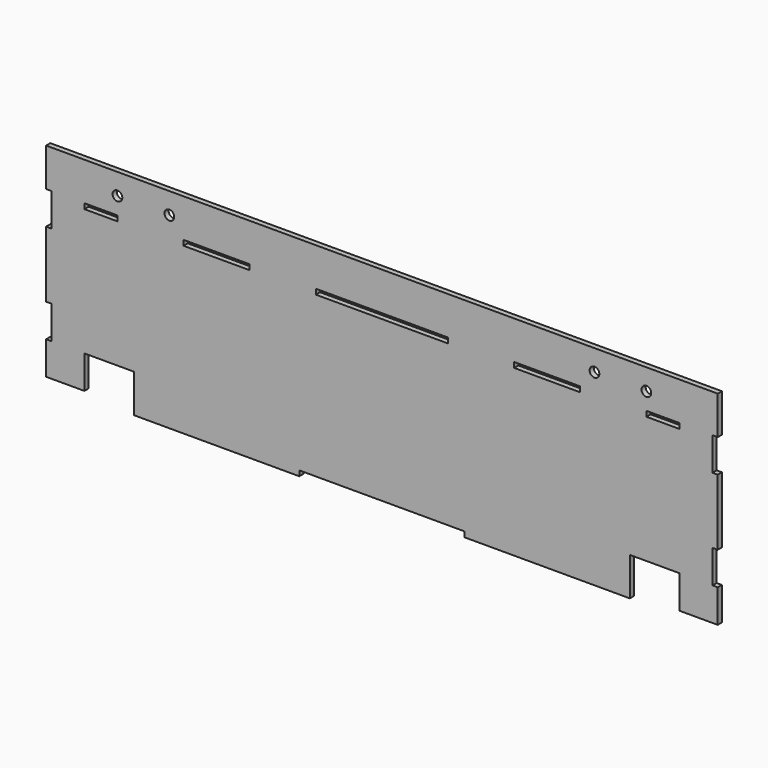
from build123d import *

# Parameters (mm, degrees)
F0_W     = 50
F0_H     = 1.5875
F0_W_2   = 1.5875
F0_H_2   = 20
F0_H_3   = 10
F0_W_3   = 10
F0_R     = 1.4732
F0_W_4   = 20
F0_W_5   = 40
F1_DEPTH = 1.5875


# Not quite as in the source:
# - a length typed as a fraction of an inch, garbled in the dataset ("3 / 203.2 mm" for 3/8 in), is restored


with BuildPart() as f1:
    # F0 (on Front) → F1 (new body)
    with BuildSketch(Plane.XZ):
        with Locations((50, -30.79375)):
            Rectangle(F0_W, F0_H)
        with Locations((-50, -30.79375)):
            Rectangle(F0_W, F0_H)
        with Locations((100.79375, 0)):
            Rectangle(F0_W_2, F0_H_2)
        with Locations((100.79375, -25)):
            Rectangle(F0_W_2, F0_H_3)
        with Locations((-100.79375, 0)):
            Rectangle(F0_W_2, F0_H_2)
        with Locations((-100.79375, -25)):
            Rectangle(F0_W_2, F0_H_3)
        with Locations((100.79375, 25)):
            Rectangle(F0_W_2, F0_H_3)
        with Locations((-100.79375, 25)):
            Rectangle(F0_W_2, F0_H_3)
        Polygon((-100, 30), (100, 30), (101.5875, 30), (101.5875, 31.5875), (-101.5875, 31.5875), (-101.5875, 30), align=None)
        Polygon((100, 20), (100, 30), (-100, 30), (-100, 20), (-100, 10), (-100, -10), (-100, -20), (-100, -30), (-90, -30), (-90, -20), (-75, -20), (-75, -30), (-25, -30), (25, -30), (75, -30), (75, -20), (90, -20), (90, -30), (100, -30), (100, -20), (100, -10), (100, 10), align=None)
        with Locations((-85, 19.20625)):
            Rectangle(F0_W_3, F0_H, mode=Mode.SUBTRACT)
        with Locations((-80, 25.1875)):
            Circle(F0_R, mode=Mode.SUBTRACT)
        with Locations((-64.3028, 25.1875)):
            Circle(F0_R, mode=Mode.SUBTRACT)
        with Locations((-50, 19.20625)):
            Rectangle(F0_W_4, F0_H, mode=Mode.SUBTRACT)
        with Locations((0, 19.20625)):
            Rectangle(F0_W_5, F0_H, mode=Mode.SUBTRACT)
        with Locations((50, 19.20625)):
            Rectangle(F0_W_4, F0_H, mode=Mode.SUBTRACT)
        with Locations((85, 19.20625)):
            Rectangle(F0_W_3, F0_H, mode=Mode.SUBTRACT)
        with Locations((64.3028, 25.1875)):
            Circle(F0_R, mode=Mode.SUBTRACT)
        with Locations((80, 25.1875)):
            Circle(F0_R, mode=Mode.SUBTRACT)
    extrude(amount=F1_DEPTH)


solid = f1.part
